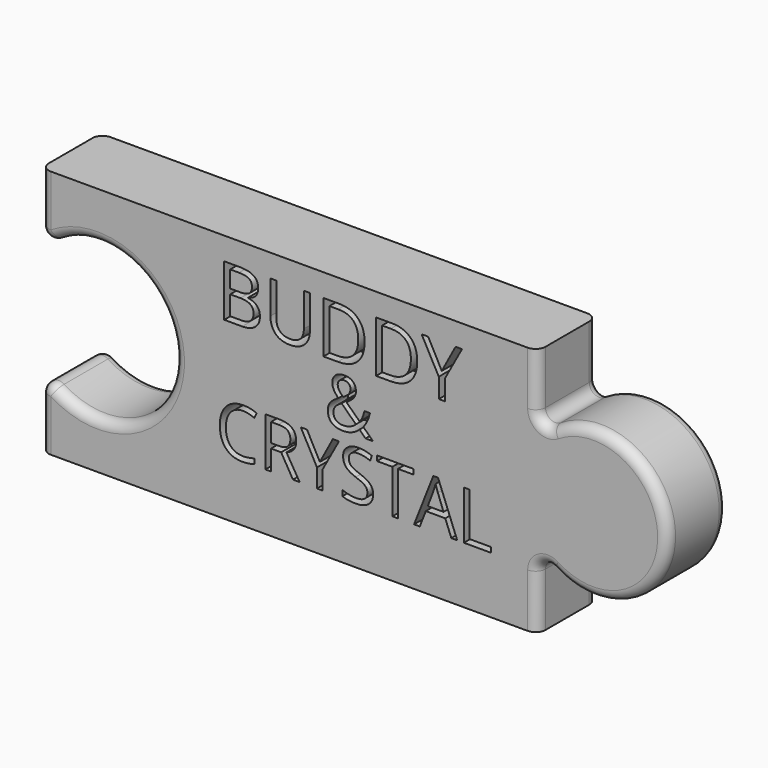
from build123d import *

# Parameters (mm, degrees)
F1_DEPTH       = 38.1
F2_F1_R        = 5.08
F2_F2_R        = 5.08
F3_TEXT_SIZE   = 36.899616114
F3_TEXT_SIZE_2 = 34.8496302548
F3_TEXT_SIZE_3 = 34.3505681182
F4_DEPTH       = 12.7


# Not quite as in the source:
# - Text() gives the source's letters only with a copy of the font that has no kerning and outlines rounded to 1/6400 em; it was checked with that copy


with BuildPart() as f1:
    # F0 (on Front) → F1 (new body)
    with BuildSketch(Plane.XZ):
        with BuildLine():
            Line((63.8834382674, 83.0045270243), (-190.1165617326, 83.0045270243))
            Line((-190.1165617326, 83.0045270243), (-190.1165617326, 45.9205270243))
            ThreePointArc((-190.1165617326, 45.9205270243), (-121.7861059351, 19.2505270243), (-190.1165617326, -7.4194729757))
            Line((-190.1165617326, -7.4194729757), (-190.1165617326, -44.5034729757))
            Line((-190.1165617326, -44.5034729757), (63.8834382674, -44.5034729757))
            Line((63.8834382674, -44.5034729757), (63.8834382674, -6.1494729757))
            ThreePointArc((63.8834382674, -6.1494729757), (130.3815015817, 19.2505270243), (63.8834382674, 44.6505270243))
            Line((63.8834382674, 44.6505270243), (63.8834382674, 83.0045270243))
        make_face()
    extrude(amount=F1_DEPTH)

    # F2: fillet of radius 5.08 on 12 edges, made by hand

    # F2_f1
    f2_f1_edges = [f1.edges().sort_by_distance(p)[0] for p in [
        (63.8834382674, -19.05, -6.1494729757),
        (63.8834382674, -19.05, 44.6505270243),
    ]]
    fillet(f2_f1_edges, radius=F2_F1_R)

    # F2_f2
    f2_f2_edges = [f1.edges().sort_by_distance(p)[0] for p in [
        (-121.7861059351, 0, 19.2505270243),
        (-190.1165617326, -19.05, 45.9205270243),
        (-190.1165617326, 0, 64.4625270243),
        (-190.1165617326, -38.1, 64.4625270243),
        (-190.1165617326, -19.05, -7.4194729757),
        (-190.1165617326, 0, -25.9614729757),
        (-190.1165617326, -38.1, -25.9614729757),
        (-121.7861059351, -38.1, 19.2505270243),
        (130.3815015817, 0, 19.2505270243),
        (130.3815015817, -38.1, 19.2505270243),
        (66.5272087993, -38.1, -12.6343036388),
        (66.5272087993, -38.1, 51.1353576873),
        (66.5272087993, 0, -12.6343036388),
        (66.5272087993, 0, 51.1353576873),
    ]]
    fillet(f2_f2_edges, radius=F2_F2_R)

    # F3 (on face) → F4 (cut)
    with BuildSketch(Plane.XZ.offset(38.1)):
        with Locations((-100.0033514574, 45.0774841011)):
            Text('BUDDY', F3_TEXT_SIZE, font='Open Sans', text_align=(TextAlign.LEFT, TextAlign.BOTTOM))
        with Locations((-100.7413566113, -15.4378740117)):
            Text('CRYSTAL', F3_TEXT_SIZE_2, font='Open Sans', text_align=(TextAlign.LEFT, TextAlign.BOTTOM))
        with Locations((-45.2746078372, 15.1602942497)):
            Text('&', F3_TEXT_SIZE_3, font='Open Sans', text_align=(TextAlign.LEFT, TextAlign.BOTTOM))
    extrude(amount=-F4_DEPTH, mode=Mode.SUBTRACT)


solid = f1.part
